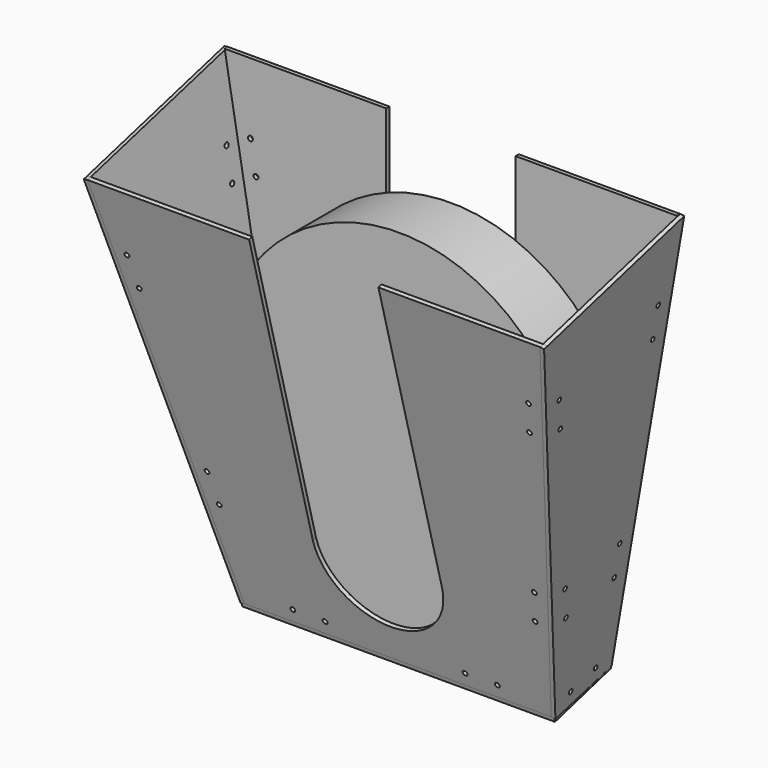
from build123d import *

# Parameters (mm, degrees)
F2_DEPTH  = 3.175
F3_R      = 139.7
F4_DEPTH  = 50.8
F8_DEPTH  = 3.175
F10_DEPTH = 3.175
F12_W     = 245.7978874445
F12_H     = 57.0418144985
F13_DEPTH = 3.175
F14_R     = 1.905
F15_DEPTH = 3.175
F16_R     = 1.905
F17_DEPTH = 362.430062838
F20_R     = 1.905
F21_DEPTH = 3.175
F22_R     = 1.905
F23_DEPTH = 3.175
F25_DEPTH = 143.0995662429


with BuildPart() as f2:
    # F1 (on Front) → F2 (new body)
    with BuildSketch(Plane.XZ):
        Polygon((120.65, 266.7), (177.8, 596.9), (-177.8, 596.9), (-120.65, 266.7), align=None)
    extrude(amount=-F2_DEPTH)

    # F20 (on face) → F21 (cut, through all)
    with BuildSketch(Plane.XZ):
        with Locations((-157.56370177, 541.3533633243)):
            Circle(F20_R)
        with Locations((-153.2319493539, 516.3254604756)):
            Circle(F20_R)
        with Locations((-126.9838096234, 364.6695420328)):
            Circle(F20_R)
        with Locations((-122.6520572073, 339.641639184)):
            Circle(F20_R)
        with Locations((-55.0182062805, 277.9206855015)):
            Circle(F20_R)
        with Locations((-80.4182062805, 277.9206855015)):
            Circle(F20_R)
        with Locations((126.9838096234, 364.6695420328)):
            Circle(F20_R)
        with Locations((153.2319493539, 516.3254604756)):
            Circle(F20_R)
        with Locations((157.56370177, 541.3533633243)):
            Circle(F20_R)
        with Locations((122.6520572073, 339.641639184)):
            Circle(F20_R)
        with Locations((55.0182062805, 277.9206855015)):
            Circle(F20_R)
        with Locations((80.4182062805, 277.9206855015)):
            Circle(F20_R)
    extrude(amount=-F21_DEPTH, mode=Mode.SUBTRACT)


with BuildPart() as f4:
    # F3 (on face) → F4 (new body)
    with BuildSketch(Plane.XZ):
        with Locations((0, 408.4407389164)):
            Circle(F3_R)
    extrude(amount=F4_DEPTH)


with BuildPart() as f8:
    # F7 (on face) → F8 (new body)
    with BuildSketch(Plane(origin=(0, 14.539153526, 3.8957544459), x_dir=(-1, 0, 0), z_dir=(0, 0.9659258263, 0.2588190451))):
        Polygon((120.65, 257.6124178713), (177.8, 576.5611257119), (-177.8, 576.5611257119), (-120.65, 257.6124178713), align=None)
    extrude(amount=F8_DEPTH)

    # F14 (on face) → F15 (cut, through all)
    with BuildSketch(Plane(origin=(0, 14.539153526, 3.8957544459), x_dir=(1, 0, 0), z_dir=(0, -0.9659258263, -0.2588190451))):
        with Locations((-157.833987404, 523.6378375606)):
            Circle(F14_R)
        with Locations((-153.3541022377, 498.6360250484)):
            Circle(F14_R)
        with Locations((-128.6446309343, 360.7348186858)):
            Circle(F14_R)
        with Locations((-124.164745768, 335.7330061736)):
            Circle(F14_R)
        with Locations((-80.4182062805, 267.9311678713)):
            Circle(F14_R)
        with Locations((-55.0182062805, 267.9311678713)):
            Circle(F14_R)
        with Locations((128.6446309343, 360.7348186858)):
            Circle(F14_R)
        with Locations((157.833987404, 523.6378375606)):
            Circle(F14_R)
        with Locations((55.0182062805, 267.9311678713)):
            Circle(F14_R)
        with Locations((124.164745768, 335.7330061736)):
            Circle(F14_R)
        with Locations((153.3541022377, 498.6360250484)):
            Circle(F14_R)
        with Locations((80.4182062805, 267.9311678713)):
            Circle(F14_R)
    extrude(amount=-F15_DEPTH, mode=Mode.SUBTRACT)


with BuildPart() as f10:
    # F9 (on face) → F10 (new body)
    with BuildSketch(Plane(origin=(-72.1731684636, 3.347089997, -12.4915099264), x_dir=(-0.0449800713, -0.99895755, -0.0077850123), z_dir=(-0.9843233273, 0.0456488032, -0.1703636528))):
        Polygon((135.102368204, 583.7099916129), (0.1788925906, 618.477983858), (0.1788925906, 283.3688038882), (52.4708201773, 270.4134080558), align=None)
        Polygon((138.1769790582, 582.9177051272), (135.102368204, 583.7099916129), (52.4708201773, 270.4134080558), (55.5408350126, 269.6036958163), align=None)
    extrude(amount=F10_DEPTH)


with BuildPart() as f11_1:
    # F11: instance of F10
    add(f10.part.mirror(Plane.YZ))


with BuildPart() as f13:
    # F12 (on face) → F13 (new body)
    with BuildSketch(Plane(origin=(0, -66.675, 248.8344875947), x_dir=(1, 0, 0), z_dir=(0, 0.2588190451, -0.9659258263))):
        with Locations((0, -43.5729465781)):
            Rectangle(F12_W, F12_H)
    extrude(amount=F13_DEPTH)

    # F22 (on face) → F23 (cut, through all)
    with BuildSketch(Plane(origin=(0, -65.8532495318, 245.7676730962), x_dir=(1, 0, 0), z_dir=(0, 0.2588190451, -0.9659258263))):
        with Locations((-80.4182062805, -28.5457893288)):
            Circle(F22_R)
        with Locations((-55.0182062805, -28.5457893288)):
            Circle(F22_R)
        with Locations((-80.4182062805, -58.6001038273)):
            Circle(F22_R)
        with Locations((-55.0182062805, -58.6001038273)):
            Circle(F22_R)
        with Locations((-109.4051937222, -30.9270393288)):
            Circle(F22_R)
        with Locations((-109.4051937222, -56.3270393288)):
            Circle(F22_R)
        with Locations((109.4051937222, -30.9270393288)):
            Circle(F22_R)
        with Locations((80.4182062805, -58.6001038273)):
            Circle(F22_R)
        with Locations((55.0182062805, -58.6001038273)):
            Circle(F22_R)
        with Locations((55.0182062805, -28.5457893288)):
            Circle(F22_R)
        with Locations((109.4051937222, -56.3270393288)):
            Circle(F22_R)
        with Locations((80.4182062805, -28.5457893288)):
            Circle(F22_R)
    extrude(amount=-F23_DEPTH, mode=Mode.SUBTRACT)


with BuildPart() as f10_1:
    add(f10.part)

    # F16 (on face) → F17 (cut, through all)
    with BuildSketch(Plane(origin=(-75.2983950276, 3.4920249471, -13.032414524), x_dir=(-0.0449800713, -0.99895755, -0.0077850123), z_dir=(-0.9843233273, 0.0456488032, -0.1703636528))):
        with Locations((62.2619372863, 347.9976447297)):
            Circle(F16_R)
        with Locations((68.7396352026, 372.5577634123)):
            Circle(F16_R)
        with Locations((104.4683391381, 508.022741925)):
            Circle(F16_R)
        with Locations((110.9460370543, 532.5828606076)):
            Circle(F16_R)
        with Locations((13.6726425906, 558.2292888641)):
            Circle(F16_R)
        with Locations((13.6726425906, 532.8292888641)):
            Circle(F16_R)
        with Locations((13.6726425906, 380.9833186626)):
            Circle(F16_R)
        with Locations((13.6726425906, 355.5833186626)):
            Circle(F16_R)
        with Locations((18.3760581746, 290.5391688496)):
            Circle(F16_R)
        with Locations((42.9361768572, 284.0614709334)):
            Circle(F16_R)
    extrude(amount=-F17_DEPTH, mode=Mode.SUBTRACT)


with BuildPart() as f19_1:
    # F19: instance of F10
    add(f10_1.part.mirror(Plane.YZ))


with BuildPart() as f25_tool:
    # F24 (on face) → F25 (new body, through all)
    with BuildSketch(Plane(origin=(0, 14.539153526, 3.8957544459), x_dir=(1, 0, 0), z_dir=(0, -0.9659258263, -0.2588190451))):
        with BuildLine():
            Line((50.8, 336.1832797527), (50.8, 576.5611257119))
            Line((50.8, 576.5611257119), (-50.8, 576.5611257119))
            Line((-50.8, 576.5611257119), (-50.8, 336.1832797527))
            Line((-50.8, 336.1832797527), (-50.8, 334.3554127512))
            ThreePointArc((-50.8, 334.3554127512), (0, 284.4611257119), (50.8, 334.3554127512))
            Line((50.8, 334.3554127512), (50.8, 336.1832797527))
        make_face()
        with BuildLine():
            ThreePointArc((50.8, 334.3554127512), (50.80822054, 335.269346252), (50.8, 336.1832797527))
            Line((50.8, 336.1832797527), (50.8, 334.3554127512))
        make_face()
        with BuildLine():
            Line((-50.8, 334.3554127512), (-50.8, 336.1832797527))
            ThreePointArc((-50.8, 336.1832797527), (-50.80822054, 335.269346252), (-50.8, 334.3554127512))
        make_face()
    extrude(amount=-F25_DEPTH)


with BuildPart() as f2_1:
    add(f2.part)

    # F25: cut by f25_tool
    add(f25_tool.part, mode=Mode.SUBTRACT)


with BuildPart() as f8_1:
    add(f8.part)

    # F25: cut by f25_tool
    add(f25_tool.part, mode=Mode.SUBTRACT)


solid = Compound([f4.part, f13.part, f10_1.part, f19_1.part, f2_1.part, f8_1.part])
